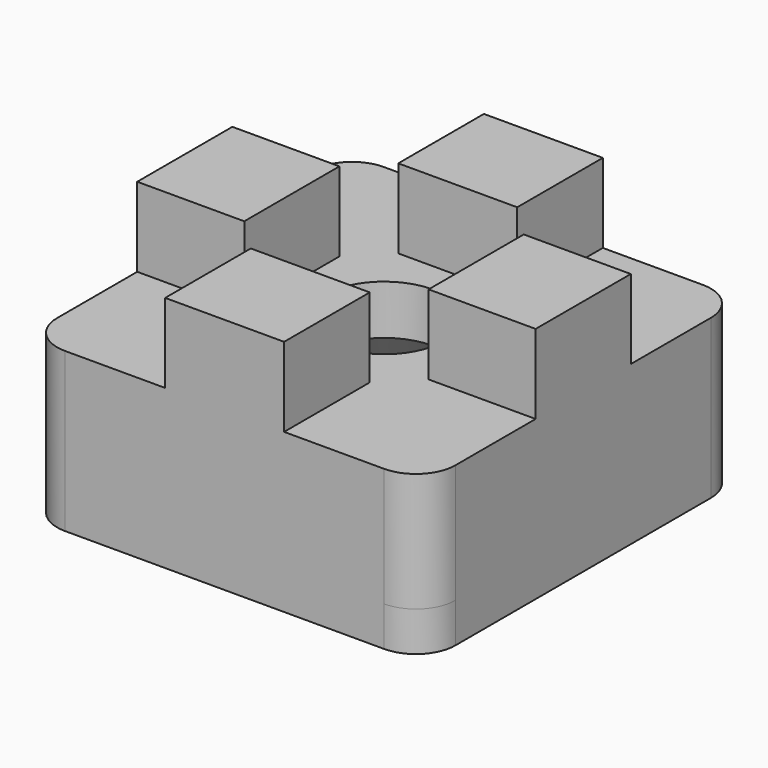
from build123d import *

# Parameters (mm, degrees)
F0_R     = 3.1
F0_W     = 5.4
F0_H     = 6
F0_W_2   = 6
F0_H_2   = 5.4
F1_DEPTH = 6
F2_DEPTH = 10
F3_R     = 2
F4_SIZE  = 3.5
F5_DEPTH = 2


# Not quite as in the source:
# - a feature names something its author has since deleted; it is built from what else it names


with BuildPart() as f1:
    # F0 (on Top) → F1 (new body)
    with BuildSketch(Plane.XY):
        Polygon((-7.9959459106, 7.05), (-7.9959459106, 0), (-0.9459459106, 0), (-0.9459459106, 5.4), (5.0540540894, 5.4), (5.0540540894, 0), (12.1040540894, 0), (12.1040540894, 7.05), (6.7040540894, 7.05), (6.7040540894, 13.05), (12.1040540894, 13.05), (12.1040540894, 20.1), (5.0540540894, 20.1), (5.0540540894, 14.7), (-0.9459459106, 14.7), (-0.9459459106, 20.1), (-7.9959459106, 20.1), (-7.9959459106, 13.05), (-2.5959459106, 13.05), (-2.5959459106, 7.05), align=None)
        with Locations((2.0540540894, 10.05)):
            Circle(F0_R, mode=Mode.SUBTRACT)
        with Locations((9.4040540894, 10.05)):
            Rectangle(F0_W, F0_H)
        with Locations((-5.2959459106, 10.05)):
            Rectangle(F0_W, F0_H)
        with Locations((2.0540540894, 17.4)):
            Rectangle(F0_W_2, F0_H_2)
        with Locations((2.0540540894, 2.7)):
            Rectangle(F0_W_2, F0_H_2)
    extrude(amount=F1_DEPTH)

    # F0 (on Top) → F2 (join)
    with BuildSketch(Plane.XY):
        with Locations((2.0540540894, 17.4)):
            Rectangle(F0_W_2, F0_H_2)
        with Locations((-5.2959459106, 10.05)):
            Rectangle(F0_W, F0_H)
        with Locations((2.0540540894, 2.7)):
            Rectangle(F0_W_2, F0_H_2)
        with Locations((9.4040540894, 10.05)):
            Rectangle(F0_W, F0_H)
    extrude(amount=F2_DEPTH)

    # F3
    f3_edges = [f1.edges().sort_by_distance(p)[0] for p in [
        (-7.995946, 0, 3),
        (12.104054, 0, 3),
        (12.104054, 20.1, 3),
        (-7.995946, 20.1, 3),
    ]]
    fillet(f3_edges, radius=F3_R)

    # F4
    f4_edges = [f1.edges().sort_by_distance(p)[0] for p in [
        (-1.045946, 10.05, 0),
    ]]
    chamfer(f4_edges, length=F4_SIZE)

    # F5 (add): a face of the model
    f5_faces = [f1.faces().sort_by_distance(p)[0] for p in [
        (-4.8302028367, 10.05, 0),
    ]]
    extrude(f5_faces, amount=F5_DEPTH)


solid = f1.part
